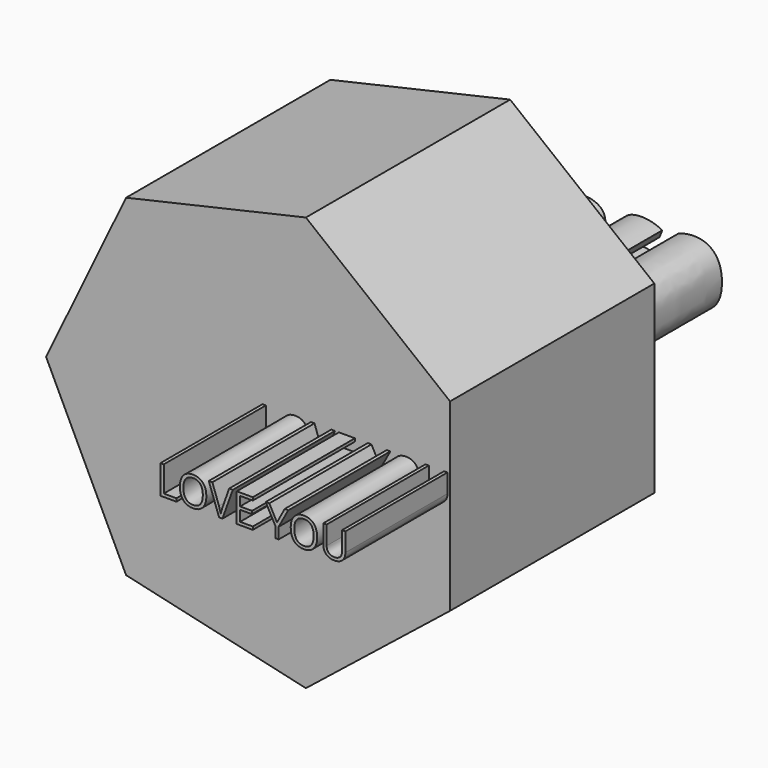
from build123d import *

# Parameters (mm, degrees)
F1_DEPTH     = 25.4
F2_TEXT_SIZE = 8.0215803671
F3_DEPTH     = 25.4
F5_DEPTH     = 25.4
F6_TEXT_SIZE = 22.5752694145
F7_DEPTH     = 25.4


# Not quite as in the source:
# - Text() gives the source's letters only with a copy of the font that has no kerning and outlines rounded to 1/6400 em; it was checked with that copy


with BuildPart() as f1:
    # F0 (on Front) → F1 (new body)
    with BuildSketch(Plane.XZ):
        Polygon((38.1, -18.3479929766), (38.1, 18.3479929766), (9.4099229016, 41.2275659875), (-26.3660180691, 33.0619409208), (-42.2878096651, 0), (-26.3660180691, -33.0619409208), (9.4099229016, -41.2275659875), align=None)
    extrude(amount=F1_DEPTH)

    # F2 (on face) → F3 (join)
    with BuildSketch(Plane.XZ.offset(25.4)):
        with Locations((0, 0)):
            Text('LOVE YOU', F2_TEXT_SIZE, font='Open Sans', text_align=(TextAlign.LEFT, TextAlign.BOTTOM))
    extrude(amount=F3_DEPTH)

    # F4 (on face) → F5 (join)
    with BuildSketch(Plane(origin=(0, 0, 0), x_dir=(-1, 0, 0), z_dir=(0, 1, 0))):
        Polygon((-38.1, -18.3479929766), (-9.4099229016, -41.2275659875), (26.3660180691, -33.0619409208), (42.2878096651, 0), (26.3660180691, 33.0619409208), (-9.4099229016, 41.2275659875), (-38.1, 18.3479929766), align=None)
    extrude(amount=F5_DEPTH)

    # F6 (on face) → F7 (join)
    with BuildSketch(Plane(origin=(0, 25.4, 0), x_dir=(-1, 0, 0), z_dir=(0, 1, 0))):
        with Locations((-32.5068525214, 0)):
            Text('cassie', F6_TEXT_SIZE, font='Open Sans', text_align=(TextAlign.LEFT, TextAlign.BOTTOM))
    extrude(amount=F7_DEPTH)


solid = f1.part
